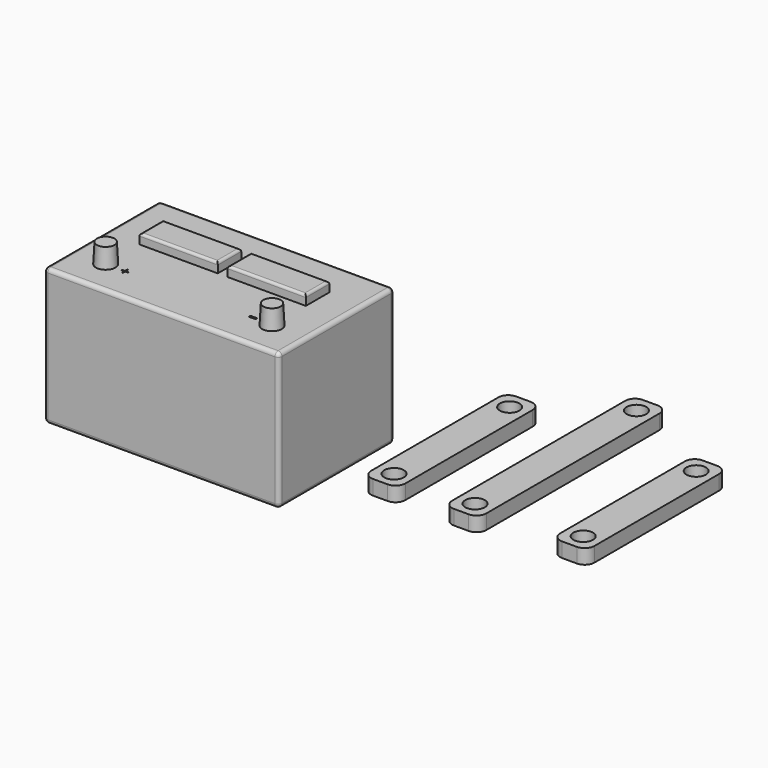
from build123d import *

# Parameters (mm, degrees)
F0_W           = 304.8
F0_H           = 177.8
F1_DEPTH       = 187.325
F2_R           = 5.08
F3_W           = 101.6
F3_H           = 38.1
F4_DEPTH       = 12.7
F3_R           = 12.7
F5_DEPTH       = 25.4
F5_TAPER       = 3
F6_R           = 3.175
F3_TEXT_SIZE   = 17.6388888889
F3_TEXT_SIZE_2 = 36.7450271248
F7_DEPTH       = 3.175
F8_R           = 12.7
F9_DEPTH       = 19.05


# Not quite as in the source:
# - Text() gives the source's letters only with a copy of the font that has no kerning and outlines rounded to 1/6400 em; it was checked with that copy


with BuildPart() as f1:
    # F0 (on Front) → F1 (new body)
    with BuildSketch(Plane.XZ):
        with Locations((-152.4, 88.9)):
            Rectangle(F0_W, F0_H)
    extrude(amount=F1_DEPTH)

    # F2
    f2_edges = [f1.edges().sort_by_distance(p)[0] for p in [
        (-152.4, -187.325, 0),
        (0, -187.325, 88.9),
        (-152.4, -187.325, 177.8),
        (-304.8, -187.325, 88.9),
        (0, -93.6625, 177.8),
        (-304.8, -93.6625, 177.8),
        (-152.4, 0, 177.8),
        (-152.4, 0, 0),
        (0, 0, 88.9),
        (-304.8, 0, 88.9),
        (-304.8, -93.6625, 0),
        (0, -93.6625, 0),
    ]]
    fillet(f2_edges, radius=F2_R)

    # F3 (on face) → F4 (join)
    with BuildSketch(Plane.XY.offset(177.8)):
        with Locations((-209.55, -68.93208987)):
            Rectangle(F3_W, F3_H)
        with Locations((-95.25, -68.9320883274)):
            Rectangle(F3_W, F3_H)
    extrude(amount=F4_DEPTH)

    # F3 (on face) → F5 (join)
    with BuildSketch(Plane.XY.offset(177.8)):
        with Locations((-260.35, -142.875)):
            Circle(F3_R)
        with Locations((-44.45, -142.875)):
            Circle(F3_R)
    extrude(amount=F5_DEPTH, taper=F5_TAPER)

    # F6
    f6_edges = [f1.edges().sort_by_distance(p)[0] for p in [
        (-260.35, -68.93209, 190.5),
        (-209.55, -87.98209, 190.5),
        (-158.75, -68.93209, 190.5),
        (-209.55, -49.88209, 190.5),
        (-44.45, -68.932088, 190.5),
        (-95.25, -49.882088, 190.5),
        (-146.05, -68.932088, 190.5),
        (-95.25, -87.982088, 190.5),
    ]]
    fillet(f6_edges, radius=F6_R)

    # F3 (on face) → F7 (cut)
    with BuildSketch(Plane.XY.offset(177.8)):
        with Locations((-240.1079969618, -149.225)):
            Text('+', F3_TEXT_SIZE, font='Open Sans', text_align=(TextAlign.LEFT, TextAlign.BOTTOM))
        with Locations((-76.2, -151.13)):
            Text('-', F3_TEXT_SIZE_2, font='Open Sans', text_align=(TextAlign.LEFT, TextAlign.BOTTOM))
    extrude(amount=-F7_DEPTH, mode=Mode.SUBTRACT)


with BuildPart() as f9:
    # F8 (on Top) → F9 (new body)
    with BuildSketch(Plane.XY):
        with BuildLine():
            Line((74.5692093611, 128.1010865936), (55.5192093611, 128.1010865936))
            ThreePointArc((55.5192093611, 128.1010865936), (46.53895324, 124.3813427146), (42.8192093611, 115.4010865936))
            Line((42.8192093611, 115.4010865936), (42.8192093611, -91.2545834064))
            ThreePointArc((42.8192093611, -91.2545834064), (46.53895324, -100.2348395275), (55.5192093611, -103.9545834064))
            Line((55.5192093611, -103.9545834064), (74.5692093611, -103.9545834064))
            ThreePointArc((74.5692093611, -103.9545834064), (83.5494654821, -100.2348395275), (87.2692093611, -91.2545834064))
            Line((87.2692093611, -91.2545834064), (87.2692093611, 115.4010865936))
            ThreePointArc((87.2692093611, 115.4010865936), (83.5494654821, 124.3813427146), (74.5692093611, 128.1010865936))
        make_face()
        with Locations((65.0442093611, -81.7295834064)):
            Circle(F8_R, mode=Mode.SUBTRACT)
        with Locations((65.0442093611, 105.8760865936)):
            Circle(F8_R, mode=Mode.SUBTRACT)
    extrude(amount=F9_DEPTH)


with BuildPart() as f9b:
    # F8 (on Top) → F9, piece 2 (new body)
    with BuildSketch(Plane.XY):
        with BuildLine():
            Line((179.7094707489, 202.3960865936), (160.6594707489, 202.3960865936))
            ThreePointArc((160.6594707489, 202.3960865936), (151.6792146278, 198.6763427146), (147.9594707489, 189.6960865936))
            Line((147.9594707489, 189.6960865936), (147.9594707489, -91.2545834064))
            ThreePointArc((147.9594707489, -91.2545834064), (151.6792146278, -100.2348395275), (160.6594707489, -103.9545834064))
            Line((160.6594707489, -103.9545834064), (179.7094707489, -103.9545834064))
            ThreePointArc((179.7094707489, -103.9545834064), (188.68972687, -100.2348395275), (192.4094707489, -91.2545834064))
            Line((192.4094707489, -91.2545834064), (192.4094707489, 189.6960865936))
            ThreePointArc((192.4094707489, 189.6960865936), (188.68972687, 198.6763427146), (179.7094707489, 202.3960865936))
        make_face()
        with Locations((170.1844707489, -81.7295834064)):
            Circle(F8_R, mode=Mode.SUBTRACT)
        with Locations((170.1844707489, 180.1710865936)):
            Circle(F8_R, mode=Mode.SUBTRACT)
    extrude(amount=F9_DEPTH)


with BuildPart() as f9c:
    # F8 (on Top) → F9, piece 3 (new body)
    with BuildSketch(Plane.XY):
        with BuildLine():
            Line((309.9563261032, 136.5338855087), (290.9063261032, 136.5338855087))
            ThreePointArc((290.9063261032, 136.5338855087), (281.9260699821, 132.8141416298), (278.2063261032, 123.8338855087))
            Line((278.2063261032, 123.8338855087), (278.2063261032, -78.5545844913))
            ThreePointArc((278.2063261032, -78.5545844913), (281.9260699821, -87.5348406123), (290.9063261032, -91.2545844913))
            Line((290.9063261032, -91.2545844913), (309.9563261032, -91.2545844913))
            ThreePointArc((309.9563261032, -91.2545844913), (318.9365822243, -87.5348406123), (322.6563261032, -78.5545844913))
            Line((322.6563261032, -78.5545844913), (322.6563261032, 123.8338855087))
            ThreePointArc((322.6563261032, 123.8338855087), (318.9365822243, 132.8141416298), (309.9563261032, 136.5338855087))
        make_face()
        with Locations((300.4313261032, -69.0295844913)):
            Circle(F8_R, mode=Mode.SUBTRACT)
        with Locations((300.4313261032, 114.3088855087)):
            Circle(F8_R, mode=Mode.SUBTRACT)
    extrude(amount=F9_DEPTH)


solid = Compound([f1.part, f9.part, f9b.part, f9c.part])
